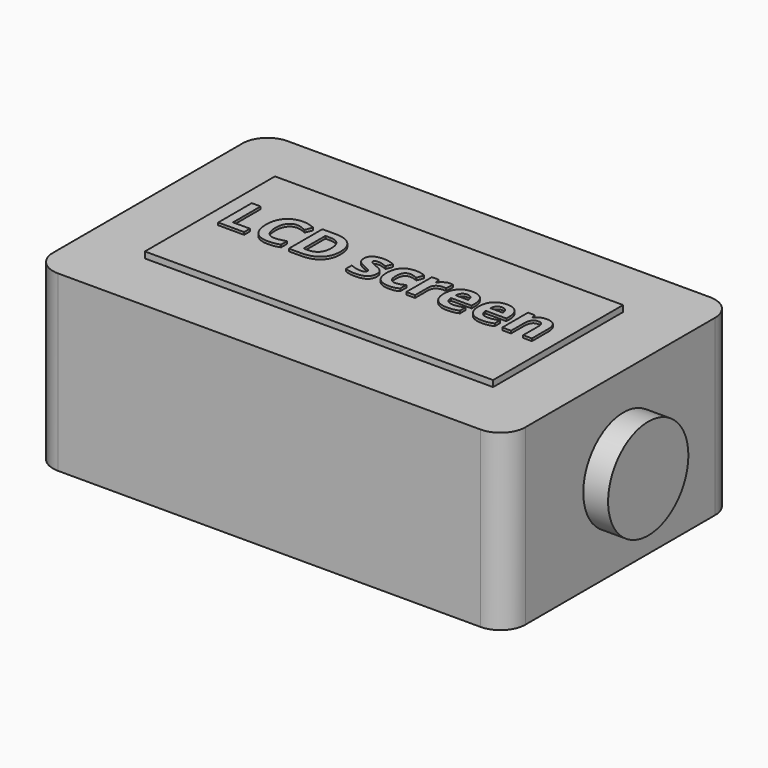
from build123d import *

# Parameters (mm, degrees)
F1_DEPTH     = 17.78
F2_W         = 35.614390704
F2_H         = 16.6269378757
F3_DEPTH     = 0.635
F4_TEXT_SIZE = 6.0079033404
F5_DEPTH     = 0.254
F6_R         = 5.1315864172
F7_DEPTH     = 2.54


# Not quite as in the source:
# - Text() gives the source's letters only with a copy of the font that has no kerning and outlines rounded to 1/6400 em; it was checked with that copy


with BuildPart() as f1:
    # F0 (on Top) → F1 (new body)
    with BuildSketch(Plane.XY):
        with BuildLine():
            Line((21.4458664572, 14.2501068926), (-21.7885242468, 14.2501068926))
            ThreePointArc((-21.7885242468, 14.2501068926), (-23.584575471, 13.5061581168), (-24.3285242468, 11.7101068926))
            Line((-24.3285242468, 11.7101068926), (-24.3285242468, -12.5368309832))
            ThreePointArc((-24.3285242468, -12.5368309832), (-23.584575471, -14.3328822074), (-21.7885242468, -15.0768309832))
            Line((-21.7885242468, -15.0768309832), (21.4458664572, -15.0768309832))
            ThreePointArc((21.4458664572, -15.0768309832), (23.2419176814, -14.3328822074), (23.9858664572, -12.5368309832))
            Line((23.9858664572, -12.5368309832), (23.9858664572, 11.7101068926))
            ThreePointArc((23.9858664572, 11.7101068926), (23.2419176814, 13.5061581168), (21.4458664572, 14.2501068926))
        make_face()
    extrude(amount=-F1_DEPTH)


with BuildPart() as f3:
    # F2 (on face) → F3 (new body, symmetric)
    with BuildSketch(Plane.XY):
        with Locations((-0.1713288948, -0.4133620453)):
            Rectangle(F2_W, F2_H)
    extrude(amount=F3_DEPTH, both=True)

    # F4 (on face) → F5 (join)
    with BuildSketch(Plane.XY.offset(0.635)):
        with Locations((-16.7698886823, -1.53776896)):
            Text('LCD screen', F4_TEXT_SIZE, font='Open Sans', font_style=FontStyle.BOLD, text_align=(TextAlign.LEFT, TextAlign.BOTTOM))
    extrude(amount=F5_DEPTH)


with BuildPart() as f7:
    # F6 (on face) → F7 (new body)
    with BuildSketch(Plane.YZ.offset(23.9858664572)):
        with Locations((0, -8.89)):
            Circle(F6_R)
    extrude(amount=F7_DEPTH)


solid = Compound([f1.part, f3.part, f7.part])
